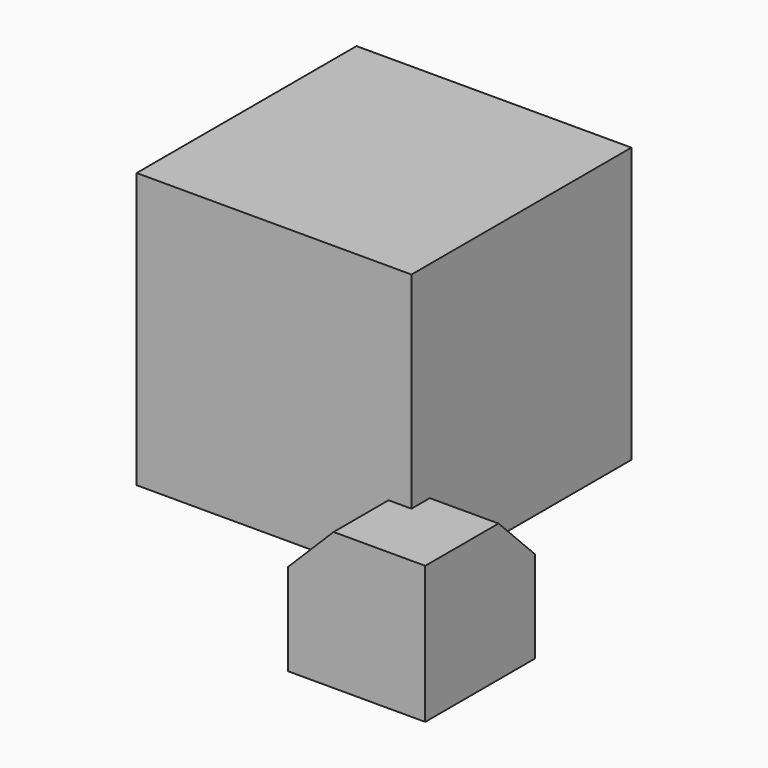
from build123d import *

# Parameters (mm, degrees)
F0_W     = 19.05
F0_H     = 19.05
F1_DEPTH = 19.05
F4_DEPTH = 9.525
F6_DEPTH = 13.8938
F8_DEPTH = 12.192


with BuildPart() as f1:
    # F0 (on Front) → F1 (new body)
    with BuildSketch(Plane.XZ):
        with Locations((9.525, 9.525)):
            Rectangle(F0_W, F0_H)
    extrude(amount=-F1_DEPTH)


with BuildPart() as f4:
    # F3 (on offset) → F4 (new body)
    with BuildSketch(Plane.XZ.offset(-4.7625)):
        Polygon((23.8125, 4.7625), (17.4625, 4.7625), (14.2875, 1.5875), (14.2875, -4.7625), (23.8125, -4.7625), align=None)
    extrude(amount=F4_DEPTH)

    # F5 (on face) → F6 (cut)
    with BuildSketch(Plane.YZ.offset(23.8125)):
        Polygon((4.7625, 4.7625), (1.5875, 4.7625), (4.7625, 1.5875), align=None)
    extrude(amount=-F6_DEPTH, mode=Mode.SUBTRACT)

    # F7 (on face) → F8 (cut)
    with BuildSketch(Plane(origin=(0, 0, -4.7625), x_dir=(1, 0, 0), z_dir=(0, 0, -1))):
        Polygon((14.2875, -1.5875), (14.2875, -4.7625), (17.4625, -4.7625), align=None)
    extrude(amount=-F8_DEPTH, mode=Mode.SUBTRACT)


solid = Compound([f1.part, f4.part])
